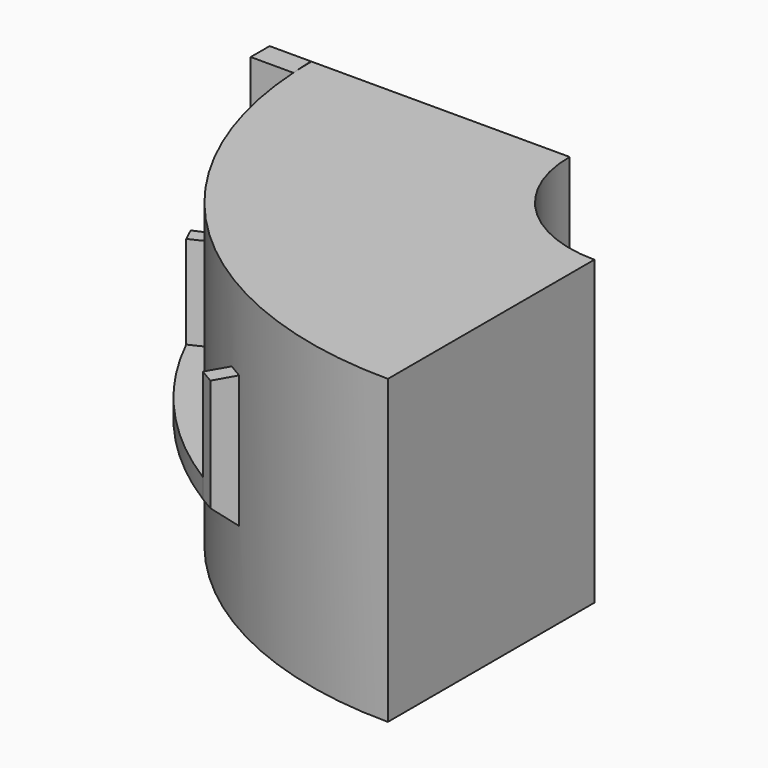
from build123d import *

# Parameters (mm, degrees)
F1_DEPTH       = 25
F4_DEPTH       = 1.6
F5_DEPTH       = 9.3
F8_ANGLE_START = 323.5
F8_ANGLE       = 36.5


# Not quite as in the source:
# - a feature names something its author has since deleted; it is built from what else it names


with BuildPart() as f1:
    # F0 (on Top) → F1 (new body)
    with BuildSketch(Plane.XY):
        Polygon((-31.6627237999, 0), (-35.0708141923, 0), (-35.0708141923, -1.9589243457), (-31.5410606563, -1.9589243457), align=None)
    extrude(amount=F1_DEPTH)


with BuildPart() as f1b:
    # F0 (on Top) → F1, piece 2 (new body)
    with BuildSketch(Plane.XY):
        with BuildLine():
            Line((-10.2362729305, 0), (-31.6018336797, 0))
            ThreePointArc((-31.6018336797, 0), (-31.5866367698, -0.97993341), (-31.5410606563, -1.9589243457))
            ThreePointArc((-31.5410606563, -1.9589243457), (-21.6422074955, -23.0280426142), (0, -31.6018336797))
            Line((0, -31.6018336797), (0, -10.2362729305))
            ThreePointArc((0, -10.2362729305), (-7.2381380033, -7.2381380033), (-10.2362729305, 0))
        make_face()
    extrude(amount=F1_DEPTH)

    # F3 (on offset) → F4 (join)
    with BuildSketch(Plane.XY.offset(9.2)):
        with BuildLine():
            Line((-28.9039363578, -12.7764766248), (-30.7331932706, -13.5850674651))
            ThreePointArc((-30.7331932706, -13.5850674651), (-30.4802346772, -14.1434974691), (-30.2171302851, -14.6972196))
            Line((-30.2171302851, -14.6972196), (-28.4130525281, -13.8338114038))
            ThreePointArc((-28.4130525281, -13.8338114038), (-28.66337023, -13.307407673), (-28.9039363578, -12.7764766248))
        make_face()
        with BuildLine():
            Line((-28.4130525281, -13.8338114038), (-30.2171302851, -14.6972196))
            ThreePointArc((-30.2171302851, -14.6972196), (-24.9696289489, -22.4855699681), (-17.771706088, -28.5175330167))
            Line((-17.771706088, -28.5175330167), (-16.7706750146, -26.7847036846))
            ThreePointArc((-16.7706750146, -26.7847036846), (-23.5015682749, -21.1270485524), (-28.4130525281, -13.8338114038))
        make_face()
        with BuildLine():
            Line((-16.7706750146, -26.7847036846), (-17.771706088, -28.5175330167))
            ThreePointArc((-17.771706088, -28.5175330167), (-17.1897915571, -28.8720330573), (-16.6008083436, -29.2146605144))
            Line((-16.6008083436, -29.2146605144), (-15.6127189136, -27.4757875236))
            ThreePointArc((-15.6127189136, -27.4757875236), (-16.1953835952, -27.1364227952), (-16.7706750146, -26.7847036846))
        make_face()
    extrude(amount=F4_DEPTH)

    # F3 (on offset) → F5 (join)
    with BuildSketch(Plane.XY.offset(9.2)):
        with BuildLine():
            Line((-16.7706750146, -26.7847036846), (-17.771706088, -28.5175330167))
            ThreePointArc((-17.771706088, -28.5175330167), (-17.1897915571, -28.8720330573), (-16.6008083436, -29.2146605144))
            Line((-16.6008083436, -29.2146605144), (-15.6127189136, -27.4757875236))
            ThreePointArc((-15.6127189136, -27.4757875236), (-16.1953835952, -27.1364227952), (-16.7706750146, -26.7847036846))
        make_face()
        with BuildLine():
            Line((-28.9039363578, -12.7764766248), (-30.7331932706, -13.5850674651))
            ThreePointArc((-30.7331932706, -13.5850674651), (-30.4802346772, -14.1434974691), (-30.2171302851, -14.6972196))
            Line((-30.2171302851, -14.6972196), (-28.4130525281, -13.8338114038))
            ThreePointArc((-28.4130525281, -13.8338114038), (-28.66337023, -13.307407673), (-28.9039363578, -12.7764766248))
        make_face()
    extrude(amount=F5_DEPTH)

    # F6 (on face) → F8 (revolve)
    with BuildSketch(Plane(origin=(0, 0, 0), x_dir=(0.494044715, 0.8694364954, 0), z_dir=(0.8694364954, -0.494044715, 0)), mode=Mode.PRIVATE) as f8_sk:
        Polygon((-31.6018336797, 9.2), (-33.6018336797, 9.2), (-31.6018336797, 7.5218007376), align=None)
    revolve(f8_sk.sketch.rotate(Axis((0, 0, 29.4944159687), (0, 0, 1)), F8_ANGLE_START), axis=Axis((0, 0, 29.4944159687), (0, 0, 1)), revolution_arc=F8_ANGLE)


solid = Compound([f1.part, f1b.part])
